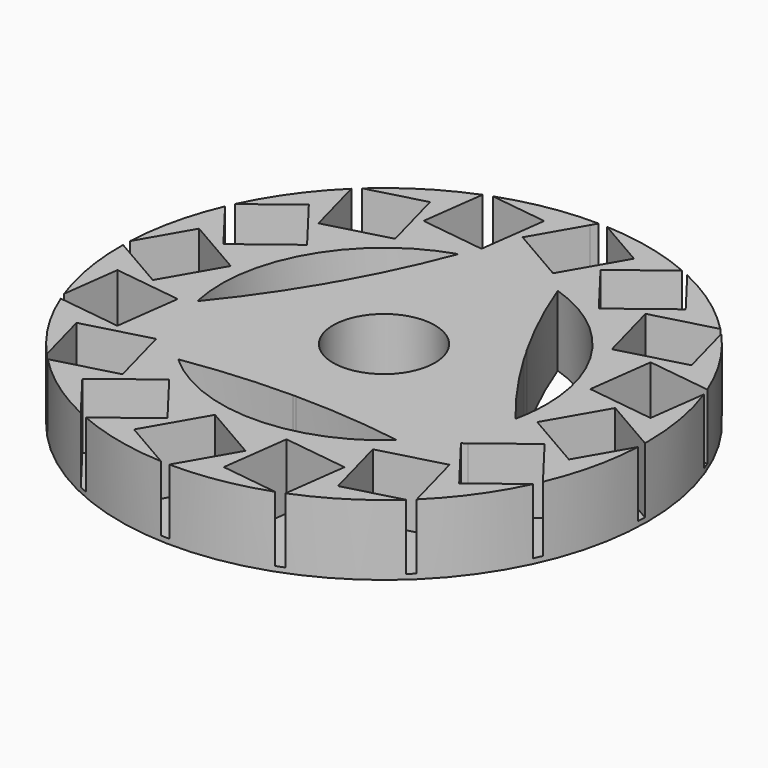
from build123d import *

# Parameters (mm, degrees)
F0_W     = 21
F0_H     = 5.6
F2_R     = 4.05
F3_DEPTH = 25
F5_DEPTH = 5.2


# Not quite as in the source:
# - a feature names something its author has since deleted; it is built from what else it names


with BuildPart() as f1:
    # F0 (on Front) → F1 (revolve)
    with BuildSketch(Plane.XZ):
        with Locations((10.5, 2.8)):
            Rectangle(F0_W, F0_H)
    revolve(axis=Axis((0, 0, 2.8), (0, 0, -1)))

    # F2 (on Top) → F3 (cut)
    with BuildSketch(Plane.XY):
        with BuildLine():
            ThreePointArc((7.42224321, 4.929341308), (7.7162863477, 4.455), (7.9800564017, 3.963180519))
            ThreePointArc((7.9800564017, 3.963180519), (10.1958256536, 0.5187206321), (12.6651471812, -2.7487536956))
            ThreePointArc((12.6651471812, -2.7487536956), (12.8860759634, -1.3822612872), (12.96, 0))
            ThreePointArc((12.96, 0), (10.4685384958, 7.640111371), (3.9520830614, 12.3427160494))
            ThreePointArc((3.9520830614, 12.3427160494), (5.5471380717, 8.5704837125), (7.42224321, 4.929341308))
        make_face()
        with BuildLine():
            ThreePointArc((8.7130641198, -9.5939623537), (4.4302657319, -9.0853125174), (0.1209660663, -8.909178818))
            ThreePointArc((0.1209660663, -8.909178818), (0, -8.91), (-0.1209660663, -8.909178818))
            ThreePointArc((-0.1209660663, -8.909178818), (-4.4302657319, -9.0853125174), (-8.7130641198, -9.5939623537))
            ThreePointArc((-8.7130641198, -9.5939623537), (0, -12.96), (8.7130641198, -9.5939623537))
        make_face()
        with BuildLine():
            ThreePointArc((-7.9723979418, 3.9785639441), (-7.7162863477, 4.455), (-7.4317364171, 4.9150171746))
            ThreePointArc((-7.4317364171, 4.9150171746), (-5.551566481, 8.5631200197), (-3.9520830614, 12.3427160494))
            ThreePointArc((-3.9520830614, 12.3427160494), (-11.223689233, 6.48), (-12.6651471812, -2.7487536956))
            ThreePointArc((-12.6651471812, -2.7487536956), (-10.1916627132, 0.5262375935), (-7.9723979418, 3.9785639441))
        make_face()
        Circle(F2_R)
    extrude(amount=F3_DEPTH, mode=Mode.SUBTRACT)

    # F4 (on face) → F5 (cut)
    with BuildSketch(Plane.XY.offset(5.6)):
        with BuildLine():
            Line((0, 15.3), (2.2516660498, 14))
            Line((2.2516660498, 14), (4.9516660498, 18.6765371804))
            Line((4.9516660498, 18.6765371804), (0.9657973165, 20.9777795666))
            ThreePointArc((0.9657973165, 20.9777795666), (0.6267497357, 20.9906451728), (0.2875385478, 20.998031374))
            Line((0.2875385478, 20.998031374), (0, 20.5))
            Line((0, 20.5), (0, 15.7))
            Line((0, 15.7), (0, 15.3))
        make_face()
        Polygon((-2.2516660498, 16.6), (0, 15.3), (0, 15.7), (0, 20.5), align=None)
        with BuildLine():
            ThreePointArc((8.9201290612, 19.011346547), (8.6118133951, 19.1529807092), (8.3012496983, 19.289615171))
            Line((8.3012496983, 19.289615171), (4.2722767998, 16.1980755322))
            Line((4.2722767998, 16.1980755322), (7.4378362306, 12.0726381627))
            Line((7.4378362306, 12.0726381627), (11.7219442682, 15.3599498793))
            Line((11.7219442682, 15.3599498793), (8.9201290612, 19.011346547))
        make_face()
        with BuildLine():
            ThreePointArc((15.5164520175, 14.150608354), (15.2858065313, 14.3994485549), (15.0511708332, 14.6445299191))
            Line((15.0511708332, 14.6445299191), (10.1458042349, 13.3301409005))
            Line((10.1458042349, 13.3301409005), (11.4916632694, 8.3073266038))
            Line((11.4916632694, 8.3073266038), (16.7076627314, 9.7049494474))
            Line((16.7076627314, 9.7049494474), (15.5164520175, 14.150608354))
        make_face()
        with BuildLine():
            ThreePointArc((19.7505358111, 7.1355683146), (19.6326741894, 7.4537308895), (19.5096876479, 7.76994774))
            Line((19.5096876479, 7.76994774), (14.4747249472, 8.4328131548))
            Line((14.4747249472, 8.4328131548), (13.7959887477, 3.2772998756))
            Line((13.7959887477, 3.2772998756), (19.1497909991, 2.5724584376))
            Line((19.1497909991, 2.5724584376), (19.7505358111, 7.1355683146))
        make_face()
        with BuildLine():
            Line((18.6765371804, -4.9516660498), (20.9777795666, -0.9657973165))
            ThreePointArc((20.9777795666, -0.9657973165), (20.9906451728, -0.6267497357), (20.998031374, -0.2875385478))
            Line((20.998031374, -0.2875385478), (16.6, 2.2516660498))
            Line((16.6, 2.2516660498), (14, -2.2516660498))
            Line((14, -2.2516660498), (18.6765371804, -4.9516660498))
        make_face()
        Polygon((17.4822978668, -10.0934093795), (12.4204504984, -7.1709504387), (12.0726381627, -7.4378362306), (15.3599498793, -11.7219442682), align=None)
        with BuildLine():
            ThreePointArc((14.150608354, -15.5164520175), (14.3994485549, -15.2858065313), (14.6445299191, -15.0511708332))
            Line((14.6445299191, -15.0511708332), (13.3301409005, -10.1458042349))
            Line((13.3301409005, -10.1458042349), (8.3073266038, -11.4916632694))
            Line((8.3073266038, -11.4916632694), (9.7049494474, -16.7076627314))
            Line((9.7049494474, -16.7076627314), (14.150608354, -15.5164520175))
        make_face()
        with BuildLine():
            ThreePointArc((7.1355683146, -19.7505358111), (7.4537308895, -19.6326741894), (7.76994774, -19.5096876479))
            Line((7.76994774, -19.5096876479), (8.4328131548, -14.4747249472))
            Line((8.4328131548, -14.4747249472), (3.2772998756, -13.7959887477))
            Line((3.2772998756, -13.7959887477), (2.5724584376, -19.1497909991))
            Line((2.5724584376, -19.1497909991), (7.1355683146, -19.7505358111))
        make_face()
        with BuildLine():
            Line((-4.9516660498, -18.6765371804), (-0.9657973165, -20.9777795666))
            ThreePointArc((-0.9657973165, -20.9777795666), (-0.6267497357, -20.9906451728), (-0.2875385478, -20.998031374))
            Line((-0.2875385478, -20.998031374), (2.2516660498, -16.6))
            Line((2.2516660498, -16.6), (-2.2516660498, -14))
            Line((-2.2516660498, -14), (-4.9516660498, -18.6765371804))
        make_face()
        with BuildLine():
            Line((-11.7219442682, -15.3599498793), (-8.9201290612, -19.011346547))
            ThreePointArc((-8.9201290612, -19.011346547), (-8.6118133951, -19.1529807092), (-8.3012496983, -19.289615171))
            Line((-8.3012496983, -19.289615171), (-4.2722767998, -16.1980755322))
            Line((-4.2722767998, -16.1980755322), (-7.4378362306, -12.0726381627))
            Line((-7.4378362306, -12.0726381627), (-11.7219442682, -15.3599498793))
        make_face()
        with BuildLine():
            Line((-16.7076627314, -9.7049494474), (-15.5164520175, -14.150608354))
            ThreePointArc((-15.5164520175, -14.150608354), (-15.2858065313, -14.3994485549), (-15.0511708332, -14.6445299191))
            Line((-15.0511708332, -14.6445299191), (-10.1458042349, -13.3301409005))
            Line((-10.1458042349, -13.3301409005), (-11.4916632694, -8.3073266038))
            Line((-11.4916632694, -8.3073266038), (-16.7076627314, -9.7049494474))
        make_face()
        with BuildLine():
            ThreePointArc((-20.9777795666, 0.9657973165), (-20.9906451728, 0.6267497357), (-20.998031374, 0.2875385478))
            Line((-20.998031374, 0.2875385478), (-16.6, -2.2516660498))
            Line((-16.6, -2.2516660498), (-14, 2.2516660498))
            Line((-14, 2.2516660498), (-18.6765371804, 4.9516660498))
            Line((-18.6765371804, 4.9516660498), (-20.9777795666, 0.9657973165))
        make_face()
        with BuildLine():
            Line((-15.3599498793, 11.7219442682), (-19.011346547, 8.9201290612))
            ThreePointArc((-19.011346547, 8.9201290612), (-19.1529807092, 8.6118133951), (-19.289615171, 8.3012496983))
            Line((-19.289615171, 8.3012496983), (-16.1980755322, 4.2722767998))
            Line((-16.1980755322, 4.2722767998), (-12.0726381627, 7.4378362306))
            Line((-12.0726381627, 7.4378362306), (-15.3599498793, 11.7219442682))
        make_face()
        with BuildLine():
            Line((-9.7049494474, 16.7076627314), (-14.150608354, 15.5164520175))
            ThreePointArc((-14.150608354, 15.5164520175), (-14.3994485549, 15.2858065313), (-14.6445299191, 15.0511708332))
            Line((-14.6445299191, 15.0511708332), (-13.3301409005, 10.1458042349))
            Line((-13.3301409005, 10.1458042349), (-8.3073266038, 11.4916632694))
            Line((-8.3073266038, 11.4916632694), (-9.7049494474, 16.7076627314))
        make_face()
        with BuildLine():
            Line((-2.5724584376, 19.1497909991), (-7.1355683146, 19.7505358111))
            ThreePointArc((-7.1355683146, 19.7505358111), (-7.4537308895, 19.6326741894), (-7.76994774, 19.5096876479))
            Line((-7.76994774, 19.5096876479), (-8.4328131548, 14.4747249472))
            Line((-8.4328131548, 14.4747249472), (-3.2772998756, 13.7959887477))
            Line((-3.2772998756, 13.7959887477), (-2.5724584376, 19.1497909991))
        make_face()
        with BuildLine():
            Line((-14.5816734862, -8.4187331125), (-14.4639209508, -8.3507486545))
            Line((-14.4639209508, -8.3507486545), (-13.7959887477, -3.2772998756))
            Line((-13.7959887477, -3.2772998756), (-19.1497909991, -2.5724584376))
            Line((-19.1497909991, -2.5724584376), (-19.7505358111, -7.1355683146))
            ThreePointArc((-19.7505358111, -7.1355683146), (-19.6326741894, -7.4537308895), (-19.5096876479, -7.76994774))
            Line((-19.5096876479, -7.76994774), (-14.5816734862, -8.4187331125))
        make_face()
        Polygon((-14.4747249472, -8.4328131548), (-14.4639209508, -8.3507486545), (-14.5816734862, -8.4187331125), align=None)
        with BuildLine():
            Line((16.1980755322, -4.2722767998), (12.4204504984, -7.1709504387))
            Line((12.4204504984, -7.1709504387), (17.4822978668, -10.0934093795))
            Line((17.4822978668, -10.0934093795), (19.011346547, -8.9201290612))
            ThreePointArc((19.011346547, -8.9201290612), (19.1529807092, -8.6118133951), (19.289615171, -8.3012496983))
            Line((19.289615171, -8.3012496983), (16.1980755322, -4.2722767998))
        make_face()
    extrude(amount=-F5_DEPTH, mode=Mode.SUBTRACT)


solid = f1.part
